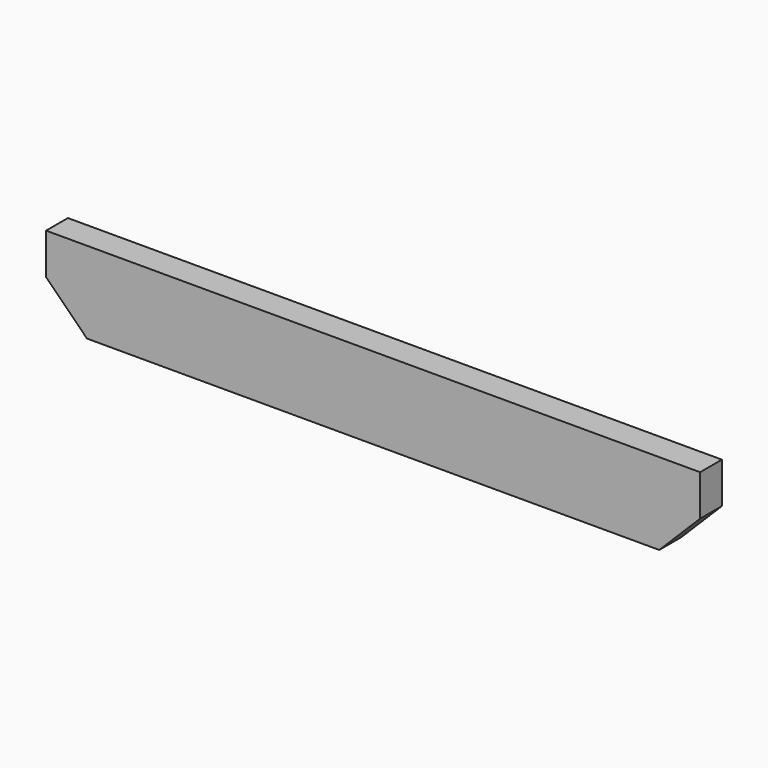
from build123d import *

# Parameters (mm, degrees)
F0_W     = 50
F0_H     = 150
F1_DEPTH = 600
F3_DEPTH = 50.001


# Not quite as in the source:
# - a pattern or mirror of a feature is missing from the dataset's text; its kind, count and spacing are read off the source's solid


with BuildPart() as f1:
    # F0 (on Right) → F1 (new body, symmetric)
    with BuildSketch(Plane.YZ):
        Rectangle(F0_W, F0_H)
    extrude(amount=F1_DEPTH, both=True)

    # F2 (on face) → F3 (cut, through all)
    with BuildSketch(Plane.XZ.offset(25)):
        Polygon((-525, -75), (-600, 0), (-600, -75), align=None)
    f3 = extrude(amount=-F3_DEPTH, mode=Mode.SUBTRACT)

    # F3_copies: F3 across plane
    add(f3.mirror(Plane(origin=(0, 0, 0), x_dir=(0, 0, 1), z_dir=(1, 0, 0))), mode=Mode.SUBTRACT)


solid = f1.part
